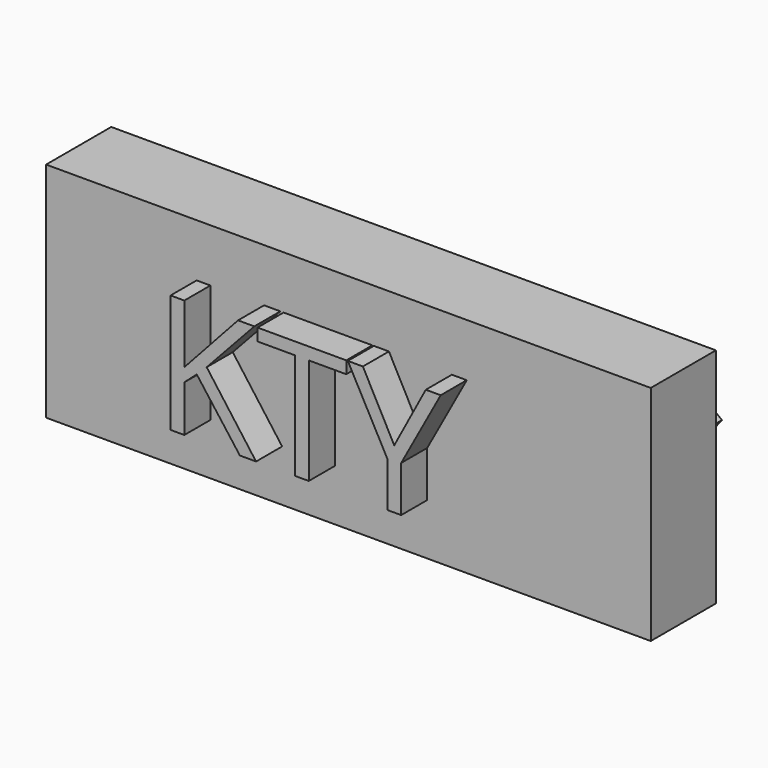
from build123d import *

# Parameters (mm, degrees)
F0_W         = 94.2974984646
F0_H         = 34.7508862615
F1_DEPTH     = 12.7
F2_TEXT_SIZE = 25.860886995
F3_DEPTH     = 5.08
F4_TEXT_SIZE = 27.3996181864
F5_DEPTH     = 4.318


# Not quite as in the source:
# - Text() gives the source's letters only with a copy of the font that has no kerning and outlines rounded to 1/6400 em; it was checked with that copy


with BuildPart() as f1:
    # F0 (on Front) → F1 (new body)
    with BuildSketch(Plane.XZ):
        with Locations((47.1487492323, 17.3754431307)):
            Rectangle(F0_W, F0_H)
    extrude(amount=F1_DEPTH)

    # F2 (on face) → F3 (join)
    with BuildSketch(Plane.XZ.offset(12.7)):
        with Locations((20.9396397695, 8.0194361508)):
            Text('KTY', F2_TEXT_SIZE, font='Open Sans', text_align=(TextAlign.LEFT, TextAlign.BOTTOM))
    extrude(amount=F3_DEPTH)

    # F4 (on face) → F5 (join)
    with BuildSketch(Plane(origin=(0, 0, 0), x_dir=(-1, 0, 0), z_dir=(0, 1, 0))):
        with Locations((-94.2974984646, 7.0441606857)):
            Text('122352', F4_TEXT_SIZE, font='Open Sans', text_align=(TextAlign.LEFT, TextAlign.BOTTOM))
    extrude(amount=F5_DEPTH)


solid = f1.part
